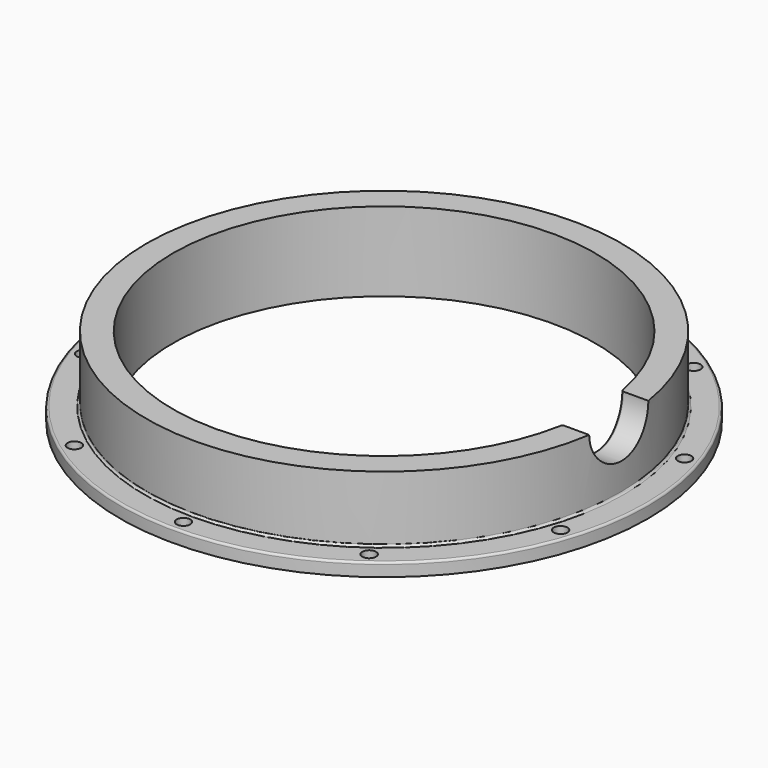
from build123d import *

# Parameters (mm, degrees)
F0_R      = 63.5
F1_DEPTH  = 3.175
F2_R      = 57.15
F3_DEPTH  = 58.7375
F4_R      = 50.8
F5_DEPTH  = 50.8
F6_R      = 1.6383
F7_DEPTH  = 3.175
F8_R      = 1.1303
F9_DEPTH  = 5.55625
F10_R     = 8.89
F11_REACH = 88.645717139
F12_R     = 0.508
F13_W     = 139.7
F13_H     = 50.8
F14_DEPTH = 63.5


with BuildPart() as f1:
    # F0 (on Top) → F1 (new body)
    with BuildSketch(Plane.XY):
        Circle(F0_R)
    extrude(amount=F1_DEPTH)

    # F2 (on Top) → F3 (join)
    with BuildSketch(Plane.XY):
        Circle(F2_R)
    extrude(amount=F3_DEPTH)

    # F4 (on face) → F5 (cut)
    with BuildSketch(Plane(origin=(0, 0, 0), x_dir=(1, 0, 0), z_dir=(0, 0, -1))):
        Circle(F4_R)
    extrude(amount=-F5_DEPTH, mode=Mode.SUBTRACT)

    # F6 (on face) → F7 (cut, through all)
    with BuildSketch(Plane(origin=(0, 0, 0), x_dir=(1, 0, 0), z_dir=(0, 0, -1))):
        with Locations((0, -60.325)):
            Circle(F6_R)
        with Locations((35.4581453445, -48.8039501857)):
            Circle(F6_R)
        with Locations((57.3724843455, -18.6414501857)):
            Circle(F6_R)
        with Locations((57.3724843455, 18.6414501857)):
            Circle(F6_R)
        with Locations((35.4581453445, 48.8039501857)):
            Circle(F6_R)
        with Locations((0, 60.325)):
            Circle(F6_R)
        with Locations((-35.4581453445, 48.8039501857)):
            Circle(F6_R)
        with Locations((-57.3724843455, 18.6414501857)):
            Circle(F6_R)
        with Locations((-57.3724843455, -18.6414501857)):
            Circle(F6_R)
        with Locations((-35.4581453445, -48.8039501857)):
            Circle(F6_R)
    extrude(amount=-F7_DEPTH, mode=Mode.SUBTRACT)

    # F8 (on face) → F9 (cut)
    with BuildSketch(Plane(origin=(0, 0, 50.8), x_dir=(1, 0, 0), z_dir=(0, 0, -1))):
        with Locations((31.115, -31.115)):
            Circle(F8_R)
        with Locations((-31.115, -31.115)):
            Circle(F8_R)
        with Locations((-31.115, 31.115)):
            Circle(F8_R)
        with Locations((31.115, 31.115)):
            Circle(F8_R)
        with Locations((31.115, 0)):
            Circle(F8_R)
        with Locations((-31.115, 0)):
            Circle(F8_R)
    extrude(amount=-F9_DEPTH, mode=Mode.SUBTRACT)

    f11_end = f1.faces().sort_by_distance((-57.15, 0, 30.95625))[0]
    # F10 (on Right) → F11 (cut, up to a face of the model that its end follows)
    with BuildSketch(Plane.YZ):
        with Locations((0, 19.05)):
            Circle(F10_R)
    f11_long = extrude(amount=F11_REACH, mode=Mode.PRIVATE)
    add(split(f11_long, bisect_by=f11_end, keep=Keep.BOTTOM, mode=Mode.PRIVATE), mode=Mode.SUBTRACT)

    # F12
    f12_edges = [f1.edges().sort_by_distance(p)[0] for p in [
        (-57.15, 0, 58.7375),
        (-63.5, 0, 3.175),
        (-57.15, 0, 3.175),
        (50.345599, 6.779427, 13.29922),
        (50.016076, -8.89, 19.051457),
    ]]
    fillet(f12_edges, radius=F12_R)

    # F13 (on Front) → F14 (cut, symmetric)
    with BuildSketch(Plane.XZ):
        with Locations((0, 44.45)):
            Rectangle(F13_W, F13_H)
    extrude(amount=F14_DEPTH, both=True, mode=Mode.SUBTRACT)


solid = f1.part
